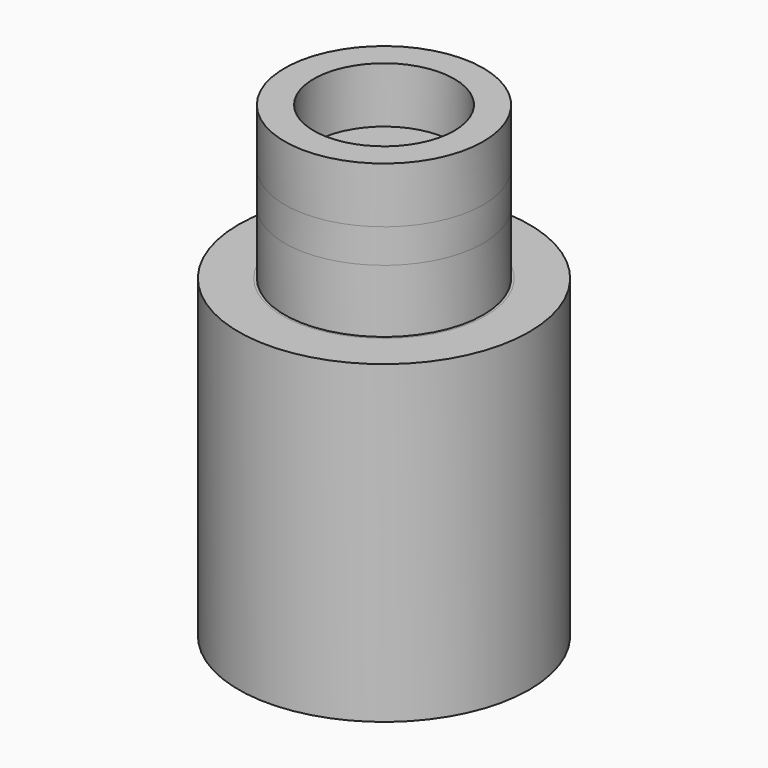
from build123d import *

# Parameters (mm, degrees)
F0_R        = 6
F0_R_2      = 4.2
F1_DEPTH    = 13
F2_R        = 4.1
F2_R_2      = 2.9
F3_DEPTH    = 6.3
F4_R        = 4.2
F4_R_2      = 2.9
F5_DEPTH    = 3
F6_S5_R     = 4.2
F6_T6_DEPTH = 9
F7_SIZE     = 0.8
F9_R        = 4.1
F10_DEPTH   = 0.7


# Not quite as in the source:
# - a fillet or chamfer that OpenCascade refuses, or shapes differently, is made with other operations: its cross-section is extruded or revolved along the edge and cut away or added


with BuildPart() as f1:
    # F0 (on Top) → F1 (new body)
    with BuildSketch(Plane.XY):
        Circle(F0_R)
        Circle(F0_R_2, mode=Mode.SUBTRACT)
    extrude(amount=F1_DEPTH)



with BuildPart() as f3:
    # F2 (on face) → F3 (new body)
    with BuildSketch(Plane.XY.offset(13)):
        Circle(F2_R)
        Circle(F2_R_2, mode=Mode.SUBTRACT)
    extrude(amount=F3_DEPTH)


with BuildPart() as f1_1:
    add(f1.part)

    add(f3.part)  # F5 merges F3
    # F4 (on face) → F5 (join)
    with BuildSketch(Plane.XY.offset(13)):
        Circle(F4_R)
        Circle(F4_R_2, mode=Mode.SUBTRACT)
    extrude(amount=-F5_DEPTH)

    # F6: chamfer of 2 on 1 edges, made by hand


with BuildPart() as f6_tool2:
    # F6_s3 → F6_t4 (revolve)
    with BuildSketch(Plane.XZ):
        Polygon((2.9, 12), (4.9, 10), (2.9, 10), align=None)
    revolve(axis=Axis((0, 0, 10), (0, 0, 1)))

    # F6_s5 → F6_t6 (intersect, symmetric)
    with BuildSketch(Plane.XY.offset(11)):
        Circle(F6_S5_R)
    extrude(amount=F6_T6_DEPTH, both=True, mode=Mode.INTERSECT)


with BuildPart() as f1_2:
    add(f1_1.part)

    # F6_t1: cut F6_tool2
    add(f6_tool2.part, mode=Mode.SUBTRACT)

    # F7
    f7_edges = [f1_2.edges().sort_by_distance(p)[0] for p in [
        (-4.2, 0, 0),
    ]]
    chamfer(f7_edges, length=F7_SIZE)

    # F9 (on offset) → F10 (join, symmetric)
    with BuildSketch(Plane.XY.offset(16.3)):
        Circle(F9_R)
    extrude(amount=F10_DEPTH, both=True)


solid = f1_2.part
